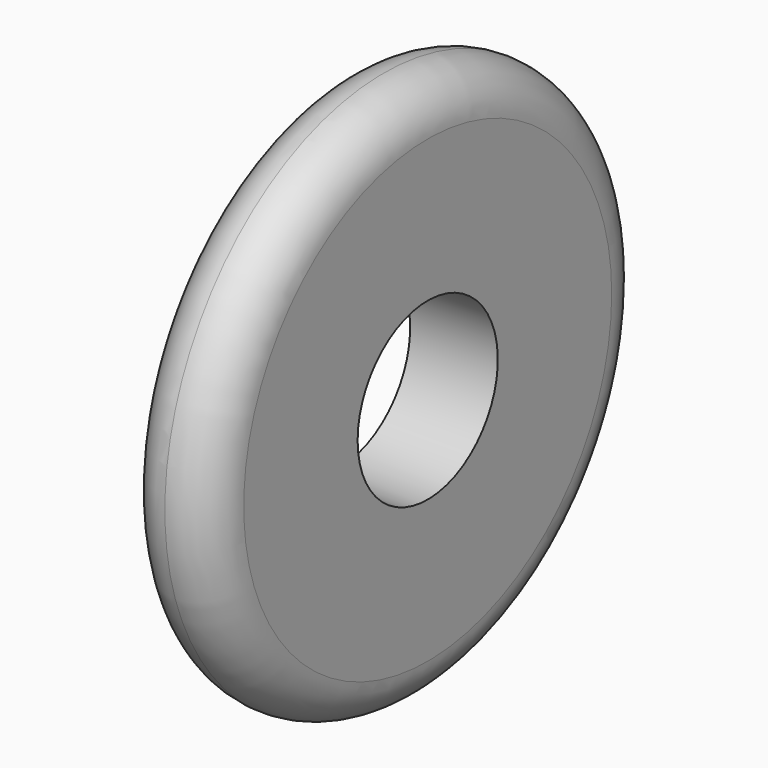
from build123d import *

# Parameters (mm, degrees)
F0_R     = 31.75
F2_DEPTH = 10.16
F3_D     = 20.32
F4_R     = 5.08
F5_R     = 5.07999


# Not quite as in the source:
# - a fillet or chamfer is up to 0.001 mm smaller than in the source, because OpenCascade refuses the exact size


with BuildPart() as f2:
    # F0 (on Right) → F2 (new body)
    with BuildSketch(Plane.YZ):
        Circle(F0_R)
    extrude(amount=F2_DEPTH)

    # F3 (through all)
    with Locations(Plane(origin=(0, 0, 0), x_dir=(0, 1, 0), z_dir=(-1, 0, 0))):
        with Locations((0, 0)):
            Hole(F3_D / 2)

    # F4
    f4_edges = [f2.edges().sort_by_distance(p)[0] for p in [
        (0, -31.75, 0),
    ]]
    fillet(f4_edges, radius=F4_R)

    # F5 (radius 5.08 in the source; OpenCascade refuses exactly that, so slightly less here)
    f5_edges = [f2.edges().sort_by_distance(p)[0] for p in [
        (10.16, -31.75, 0),
    ]]
    fillet(f5_edges, radius=F5_R)


solid = f2.part
